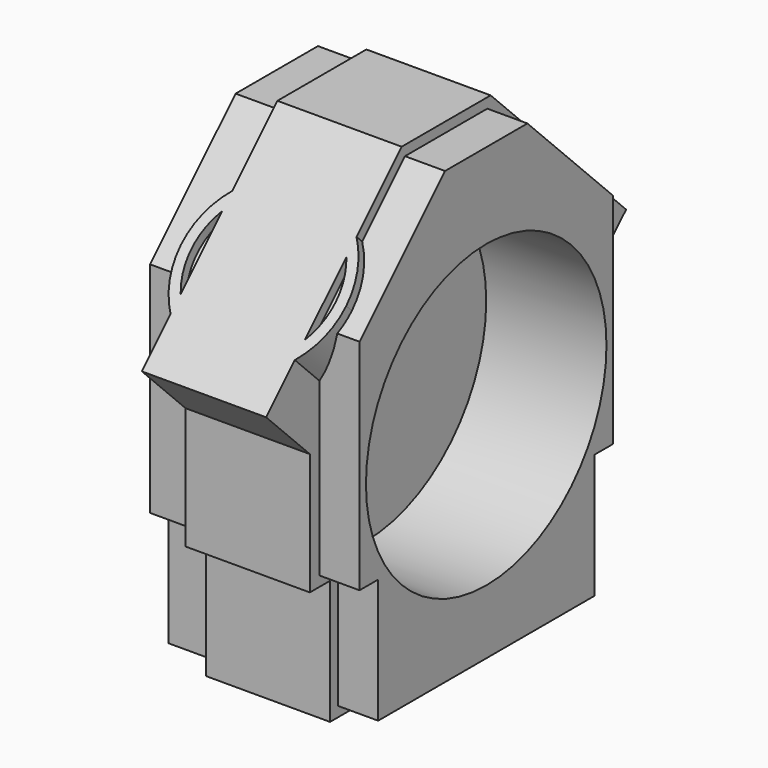
from build123d import *

# Parameters (mm, degrees)
F0_R     = 15
F1_DEPTH = 124
F3_DEPTH = 40
F4_R     = 15
F5_DEPTH = 45
F7_DEPTH = 100
F8_R     = 150
F8_R_2   = 15
F9_DEPTH = 120


with BuildPart() as f1:
    # F0 (on Right) → F1 (new body)
    with BuildSketch(Plane.YZ):
        Polygon((-55.507882, 234.50625), (-150.260191, 139.753941), (-224.506403, 65.507729), (-170, 11.001326), (-170, -110.50625), (-144.782609, -110.50625), (-144.782609, -234.50625), (144.782609, -234.50625), (144.782609, -110.50625), (170, -110.50625), (170, 11.001326), (224.506403, 65.507729), (150.260191, 139.753941), (55.507882, 234.50625), align=None)
        with Locations((0, -10.50625)):
            Circle(F0_R, mode=Mode.SUBTRACT)
    extrude(amount=F1_DEPTH)

    # F2 (on face) → F3 (join)
    with BuildSketch(Plane.YZ.offset(124)):
        Polygon((0, 224.50625), (-51.3657463763, 224.50625), (-158, 117.8719963763), (-158, -100.50625), (-134.782609, -100.50625), (-134.782609, -224.50625), (0, -224.50625), (134.782609, -224.50625), (134.782609, -100.50625), (158, -100.50625), (158, 117.8719963763), (51.3657463763, 224.50625), align=None)
        with BuildLine():
            ThreePointArc((15, -10.50625), (-10.6066017178, -21.1128517178), (0, 4.49375))
            ThreePointArc((0, 4.49375), (10.6066017178, 0.1003517178), (15, -10.50625))
        make_face(mode=Mode.SUBTRACT)
    extrude(amount=F3_DEPTH)

    # F4 (on face) → F5 (join)
    with BuildSketch(Plane(origin=(0, 0, 0), x_dir=(0, -1, 0), z_dir=(-1, 0, 0))):
        Polygon((134.782609, -100.50625), (158, -100.50625), (158, 117.8719963763), (51.3657463763, 224.50625), (0, 224.50625), (-51.3657463763, 224.50625), (-158, 117.8719963763), (-158, -100.50625), (-134.782609, -100.50625), (-134.782609, -224.50625), (0, -224.50625), (134.782609, -224.50625), align=None)
        with Locations((0, -10.50625)):
            Circle(F4_R, mode=Mode.SUBTRACT)
    extrude(amount=F5_DEPTH)

    # F6 (on face) → F7 (join)
    with BuildSketch(Plane(origin=(0, -145.007066, 145.007066), x_dir=(1, 0, 0), z_dir=(0, -0.7071067812, 0.7071067812))):
        with BuildLine():
            ThreePointArc((124, -61.8555966032), (139.2050840295, -36.5086726323), (144.5, -7.4290405851))
            ThreePointArc((144.5, -7.4290405851), (139.2050840295, 21.6505914621), (124, 46.9975154331))
            Line((124, 46.9975154331), (124, 29.1769698504))
            ThreePointArc((124, 29.1769698504), (131.4550214167, 11.5446253759), (134, -7.4290405851))
            ThreePointArc((134, -7.4290405851), (131.4550214167, -26.4027065461), (124, -44.0350510205))
            Line((124, -44.0350510205), (124, -61.8555966032))
        make_face()
        with BuildLine():
            ThreePointArc((0, -61.8555966032), (62, -89.9290405851), (124, -61.8555966032))
            Line((124, -61.8555966032), (124, -44.0350510205))
            ThreePointArc((124, -44.0350510205), (62, -79.4290405851), (0, -44.0350510205))
            Line((0, -44.0350510205), (0, -61.8555966033))
        make_face()
        with BuildLine():
            Line((0, 29.1769698504), (0, 46.9975154331))
            ThreePointArc((0, 46.9975154331), (-20.5, -7.4290405851), (0, -61.8555966032))
            Line((0, -61.8555966033), (0, -44.0350510205))
            ThreePointArc((0, -44.0350510205), (-10, -7.4290405851), (0, 29.1769698504))
        make_face()
    extrude(amount=-F7_DEPTH)

    # F8 (on face) → F9 (cut)
    with BuildSketch(Plane.YZ.offset(164)):
        with Locations((0, -10.50625)):
            Circle(F8_R)
        with Locations((0, -10.50625)):
            Circle(F8_R_2, mode=Mode.SUBTRACT)
    extrude(amount=-F9_DEPTH, mode=Mode.SUBTRACT)


solid = f1.part
